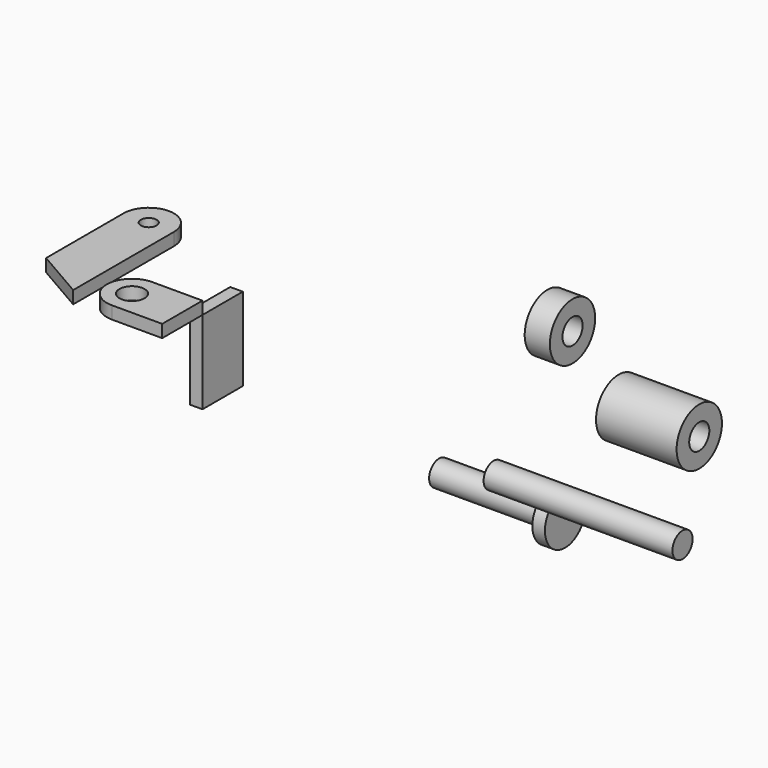
from build123d import *

# Parameters (mm, degrees)
F0_W      = 6.35
F0_H      = 41.91
F1_DEPTH  = 25.4
F3_DEPTH  = 25.4
F4_R      = 6.35
F5_DEPTH  = 6.35
F6_R      = 14.2875
F6_R_2    = 6.35
F7_DEPTH  = 12.7
F8_R      = 6.35
F9_DEPTH  = 95.25
F10_R     = 14.2875
F10_R_2   = 6.35
F11_DEPTH = 40.64
F12_R     = 12.7
F13_DEPTH = 6.35
F14_R     = 6.35
F15_DEPTH = 57.15
F16_R     = 3.96875
F17_DEPTH = 6.35
F18_R     = 12.69999


# Not quite as in the source:
# - a fillet or chamfer is up to 0.001 mm smaller than in the source, because OpenCascade refuses the exact size


with BuildPart() as f1:
    # F0 (on Front) → F1 (new body)
    with BuildSketch(Plane.XZ):
        with Locations((-84.3865873288, 23.4739605102)):
            Rectangle(F0_W, F0_H)
    extrude(amount=F1_DEPTH)


with BuildPart() as f3:
    # F2 (on face) → F3 (new body)
    with BuildSketch(Plane.XZ.offset(25.4)):
        Polygon((-87.5615873288, 44.4289605102), (-81.2115873288, 44.4289605102), (-81.2115873288, 50.7789605102), (-119.3115873288, 50.7789605102), (-119.3115873288, 44.4289605102), align=None)
    extrude(amount=F3_DEPTH)

    # F4 (on face) → F5 (cut, through all)
    with BuildSketch(Plane.XY.offset(50.7789605102)):
        with Locations((-106.6115873288, -38.1)):
            Circle(F4_R)
    extrude(amount=-F5_DEPTH, mode=Mode.SUBTRACT)

    # F18 (radius 12.7 in the source; OpenCascade refuses exactly that, so slightly less here)
    f18_edges = [f3.edges().sort_by_distance(p)[0] for p in [
        (-119.311587, -50.8, 47.603961),
        (-119.311587, -25.4, 47.603961),
    ]]
    fillet(f18_edges, radius=F18_R)


with BuildPart() as f7:
    # F6 (on Right) → F7 (new body)
    with BuildSketch(Plane.YZ):
        with Locations((90.4932394624, 20.6049848348)):
            Circle(F6_R)
        with Locations((90.4932394624, 20.6049848348)):
            Circle(F6_R_2, mode=Mode.SUBTRACT)
    extrude(amount=F7_DEPTH)


with BuildPart() as f9:
    # F8 (on Right) → F9 (new body)
    with BuildSketch(Plane.YZ):
        with Locations((56.6555783153, -33.6186587811)):
            Circle(F8_R)
    extrude(amount=F9_DEPTH)


with BuildPart() as f11:
    # F10 (on Right) → F11 (new body)
    with BuildSketch(Plane.YZ):
        with Locations((135.4606151581, -35.3056155145)):
            Circle(F10_R)
        with Locations((135.4606151581, -35.3056155145)):
            Circle(F10_R_2, mode=Mode.SUBTRACT)
    extrude(amount=F11_DEPTH)


with BuildPart() as f13:
    # F12 (on Right) → F13 (new body)
    with BuildSketch(Plane.YZ):
        with Locations((93.7340855598, -66.2199109793)):
            Circle(F12_R)
    extrude(amount=F13_DEPTH)

    # F14 (on face) → F15 (join)
    with BuildSketch(Plane(origin=(0, 0, 0), x_dir=(0, -1, 0), z_dir=(-1, 0, 0))):
        with Locations((-93.7340855598, -66.2199109793)):
            Circle(F14_R)
    extrude(amount=F15_DEPTH)


with BuildPart() as f17:
    # F16 (on Top) → F17 (new body)
    with BuildSketch(Plane.XY):
        with BuildLine():
            Line((-179.9224981273, 16.4599019216), (-179.9224981273, 79.9599019216))
            ThreePointArc((-179.9224981273, 79.9599019216), (-183.6422420062, 88.9401580427), (-192.6224981273, 92.6599019216))
            ThreePointArc((-192.6224981273, 92.6599019216), (-201.6027542484, 88.9401580427), (-205.3224981273, 79.9599019216))
            Line((-205.3224981273, 79.9599019216), (-205.3224981273, 31.124598759))
            Line((-205.3224981273, 31.124598759), (-179.9224981273, 16.4599019216))
        make_face()
        with Locations((-192.6224981273, 79.9599019216)):
            Circle(F16_R, mode=Mode.SUBTRACT)
    extrude(amount=F17_DEPTH)


solid = Compound([f1.part, f3.part, f7.part, f9.part, f11.part, f13.part, f17.part])
